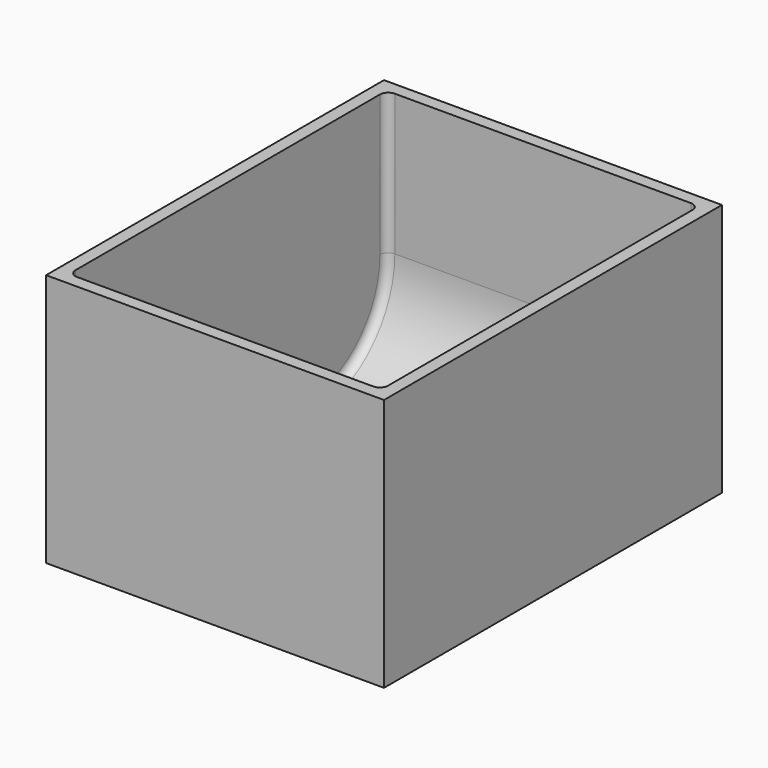
from build123d import *

# Parameters (mm, degrees)
F0_W     = 101.6
F0_H     = 127
F1_DEPTH = 76.2
F2_T     = -3.81
F3_R     = 30
F4_R     = 2.5
F5_DEPTH = 76.2


with BuildPart() as f1:
    # F0 (on Top) → F1 (new body)
    with BuildSketch(Plane.XY):
        Rectangle(F0_W, F0_H)
    extrude(amount=F1_DEPTH)

    # F2
    f2_openings = [f1.faces().sort_by_distance(p)[0] for p in [
        (0, 0, 76.2),
    ]]
    offset(amount=F2_T, openings=f2_openings)

    # F3
    f3_edges = [f1.edges().sort_by_distance(p)[0] for p in [
        (0, 59.69, 3.81),
        (0, -59.69, 3.81),
    ]]
    fillet(f3_edges, radius=F3_R)

    # F4
    f4_edges = [f1.edges().sort_by_distance(p)[0] for p in [
        (-46.99, -50.903203, 12.596797),
        (46.99, -50.903203, 12.596797),
    ]]
    fillet(f4_edges, radius=F4_R)

    # F5 (add): a face of the model
    f5_faces = [f1.faces().sort_by_distance(p)[0] for p in [
        (0, -61.3163935563, 76.2),
    ]]
    extrude(f5_faces, amount=-F5_DEPTH)


solid = f1.part
